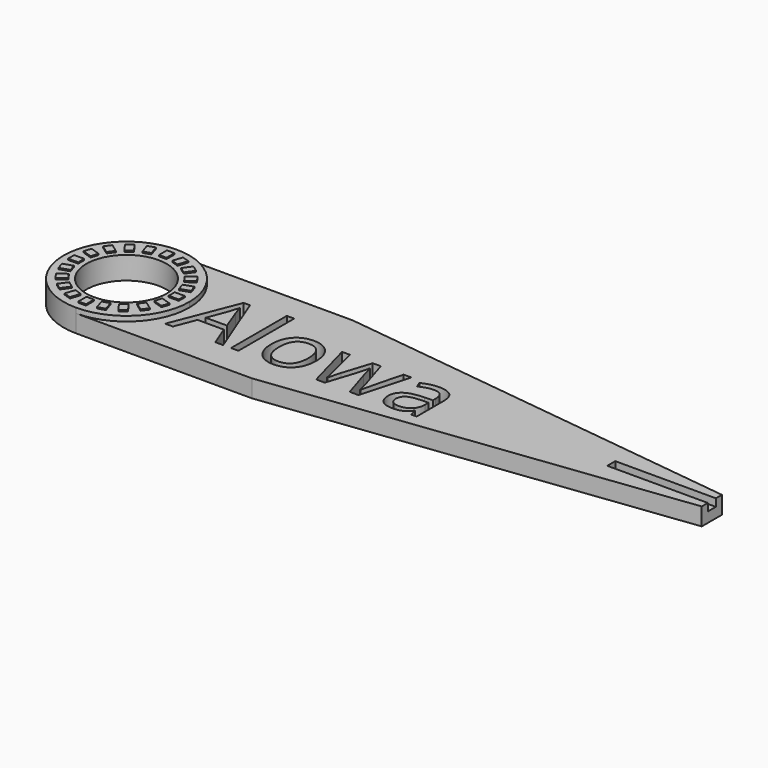
from build123d import *

# Parameters (mm, degrees)
F0_R         = 8
F1_DEPTH     = 3.5
F2_R         = 8
F3_DEPTH     = 1
F4_W         = 1.5
F4_H         = 2
F4_W_2       = 2
F4_H_2       = 1.5
F5_DEPTH     = 0.25
F6_W         = 20
F6_H         = 2
F7_DEPTH     = 1.5
F8_TEXT_SIZE = 18.229167391
F9_DEPTH     = 25


# Not quite as in the source:
# - Text() gives the source's letters only with a copy of the font that has no kerning and outlines rounded to 1/6400 em; it was checked with that copy


with BuildPart() as f1:
    # F0 (on Top) → F1 (new body)
    with BuildSketch(Plane.XY):
        with BuildLine():
            ThreePointArc((0, -12.5), (8.8388347648, -8.8388347648), (12.5, 0))
            ThreePointArc((12.5, 0), (8.8388347648, 8.8388347648), (0, 12.5))
            ThreePointArc((0, 12.5), (-12.5, 0), (0, -12.5))
        make_face()
        Circle(F0_R, mode=Mode.SUBTRACT)
        with BuildLine():
            ThreePointArc((0, 12.5), (8.8388347648, 8.8388347648), (12.5, 0))
            ThreePointArc((12.5, 0), (8.8388347648, -8.8388347648), (0, -12.5))
            Line((0, -12.5), (35, -12.5))
            Line((35, -12.5), (116.3887844346, -2.5067138408))
            Line((116.3887844346, -2.5067138408), (116.3887844346, 2.5067138408))
            Line((116.3887844346, 2.5067138408), (35, 12.5))
            Line((35, 12.5), (0, 12.5))
        make_face()
    extrude(amount=F1_DEPTH)

    # F2 (on face) → F3 (join)
    with BuildSketch(Plane.XY.offset(3.5)):
        with BuildLine():
            ThreePointArc((0, -12.5), (8.8388347648, -8.8388347648), (12.5, 0))
            ThreePointArc((12.5, 0), (8.8388347648, 8.8388347648), (0, 12.5))
            ThreePointArc((0, 12.5), (-12.5, 0), (0, -12.5))
        make_face()
        Circle(F2_R, mode=Mode.SUBTRACT)
    extrude(amount=F3_DEPTH)

    # F4 (on face) → F5 (join)
    with BuildSketch(Plane.XY.offset(4.5)):
        with Locations((0, 10)):
            Rectangle(F4_W, F4_H)
        Polygon((-2.6858945509, 10.693384425), (-4.1124793253, 10.2298589335), (-3.4944453366, 8.3277459009), (-2.0678605622, 8.7912713924), align=None)
        Polygon((-5.8588750294, 9.3400258773), (-7.072400521, 8.4583479989), (-5.8968300164, 6.8403140102), (-4.6833045249, 7.7219918886), align=None)
        Polygon((-8.4583479989, 7.072400521), (-9.3400258773, 5.8588750294), (-7.7219918886, 4.6833045249), (-6.8403140102, 5.8968300164), align=None)
        Polygon((-10.2298589335, 4.1124793253), (-10.693384425, 2.6858945509), (-8.7912713924, 2.0678605622), (-8.3277459009, 3.4944453366), align=None)
        with Locations((-10, 0)):
            Rectangle(F4_W_2, F4_H_2)
        Polygon((-10.693384425, -2.6858945509), (-10.2298589335, -4.1124793253), (-8.3277459009, -3.4944453366), (-8.7912713924, -2.0678605622), align=None)
        Polygon((-9.3400258773, -5.8588750294), (-8.4583479989, -7.072400521), (-6.8403140102, -5.8968300164), (-7.7219918886, -4.6833045249), align=None)
        Polygon((-7.072400521, -8.4583479989), (-5.8588750294, -9.3400258773), (-4.6833045249, -7.7219918886), (-5.8968300164, -6.8403140102), align=None)
        Polygon((-4.1124793253, -10.2298589335), (-2.6858945509, -10.693384425), (-2.0678605622, -8.7912713924), (-3.4944453366, -8.3277459009), align=None)
        with Locations((0, -10)):
            Rectangle(F4_W, F4_H)
        Polygon((2.6858945509, -10.693384425), (4.1124793253, -10.2298589335), (3.4944453366, -8.3277459009), (2.0678605622, -8.7912713924), align=None)
        Polygon((5.8588750294, -9.3400258773), (7.072400521, -8.4583479989), (5.8968300164, -6.8403140102), (4.6833045249, -7.7219918886), align=None)
        Polygon((8.4583479989, -7.072400521), (9.3400258773, -5.8588750294), (7.7219918886, -4.6833045249), (6.8403140102, -5.8968300164), align=None)
        Polygon((10.2298589335, -4.1124793253), (10.693384425, -2.6858945509), (8.7912713924, -2.0678605622), (8.3277459009, -3.4944453366), align=None)
        with Locations((10, 0)):
            Rectangle(F4_W_2, F4_H_2)
        Polygon((10.693384425, 2.6858945509), (10.2298589335, 4.1124793253), (8.3277459009, 3.4944453366), (8.7912713924, 2.0678605622), align=None)
        Polygon((9.3400258773, 5.8588750294), (8.4583479989, 7.072400521), (6.8403140102, 5.8968300164), (7.7219918886, 4.6833045249), align=None)
        Polygon((7.072400521, 8.4583479989), (5.8588750294, 9.3400258773), (4.6833045249, 7.7219918886), (5.8968300164, 6.8403140102), align=None)
        Polygon((4.1124793253, 10.2298589335), (2.6858945509, 10.693384425), (2.0678605622, 8.7912713924), (3.4944453366, 8.3277459009), align=None)
    extrude(amount=F5_DEPTH)

    # F6 (on face) → F7 (cut)
    with BuildSketch(Plane.XY.offset(3.5)):
        with Locations((106.3887844346, 0.0067138408)):
            Rectangle(F6_W, F6_H)
    extrude(amount=-F7_DEPTH, mode=Mode.SUBTRACT)

    # F8 (on Top) → F9 (cut)
    with BuildSketch(Plane.XY):
        with Locations((12.9387080669, -6.5625002608)):
            Text('Alowa', F8_TEXT_SIZE, font='Open Sans', text_align=(TextAlign.LEFT, TextAlign.BOTTOM))
    extrude(amount=F9_DEPTH, mode=Mode.SUBTRACT)


solid = f1.part
